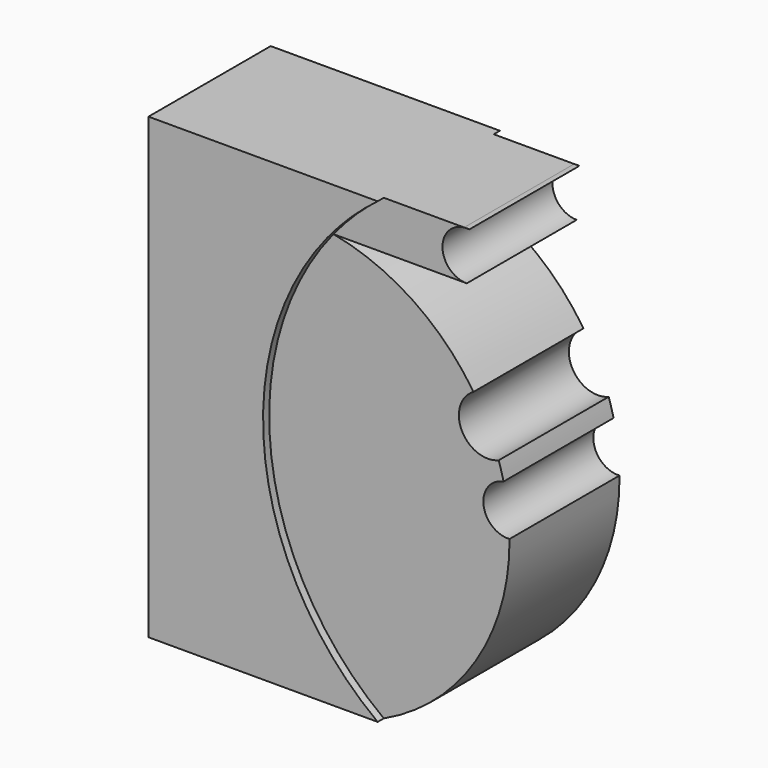
from build123d import *

# Parameters (mm, degrees)
F1_DEPTH = 25.4
F2_DEPTH = 22.86


with BuildPart() as f1:
    # F0 (on Front) → F1 (new body, symmetric)
    with BuildSketch(Plane.XZ):
        with BuildLine():
            Line((-38.1, -76.2), (38.1, -76.2))
            ThreePointArc((38.1, -76.2), (0.709542394, -11.6044980782), (21.3676740894, 60.1162575185))
            ThreePointArc((21.3676740894, 60.1162575185), (29.2421269738, 68.6696672379), (38.1, 76.2))
            Line((38.1, 76.2), (17.5172466843, 76.2))
            Line((17.5172466843, 76.2), (-38.1, 76.2))
            Line((-38.1, 76.2), (-38.1, -76.2))
        make_face()
    extrude(amount=F1_DEPTH, both=True)



with BuildPart() as f2:
    # F0 (on Front) → F2 (new body, symmetric)
    with BuildSketch(Plane.XZ):
        with BuildLine():
            ThreePointArc((66.565518939, 76.2), (65.6902864575, 76.2476277146), (64.8150539761, 76.2))
            Line((64.8150539761, 76.2), (66.565518939, 76.2))
        make_face()
    extrude(amount=F2_DEPTH, both=True)


with BuildPart() as f1_1:
    add(f1.part)

    add(f2.part)  # F2#2 merges F2
    # F0 (on Front) → F2, piece 2 (join, symmetric)
    with BuildSketch(Plane.XZ):
        with BuildLine():
            ThreePointArc((38.1, 76.2), (29.2421269738, 68.6696672379), (21.3676740894, 60.1162575185))
            Line((21.3676740894, 60.1162575185), (65.6902864575, 60.1162575185))
            ThreePointArc((65.6902864575, 60.1162575185), (57.6365170899, 67.7436789129), (64.8150539761, 76.2))
            Line((64.8150539761, 76.2), (38.1, 76.2))
        make_face()
        with BuildLine():
            ThreePointArc((21.3676740894, 60.1162575185), (0.709542394, -11.6044980782), (38.1, -76.2))
            ThreePointArc((38.1, -76.2), (68.7424455832, -49.3054294639), (79.9131497153, -10.0945538702))
            ThreePointArc((79.9131497153, -10.0945538702), (71.275473587, -2.9427861122), (77.9270839804, 6.0856860805))
            ThreePointArc((77.9270839804, 6.0856860805), (77.1783216459, 8.9480305918), (76.3128333068, 11.7772691943))
            ThreePointArc((76.3128333068, 11.7772691943), (64.037134436, 16.508200152), (67.9383126947, 29.0722480144))
            ThreePointArc((67.9383126947, 29.0722480144), (47.785974111, 49.2941905371), (21.3676740894, 60.1162575185))
        make_face()
    extrude(amount=F2_DEPTH, both=True)


solid = f1_1.part
